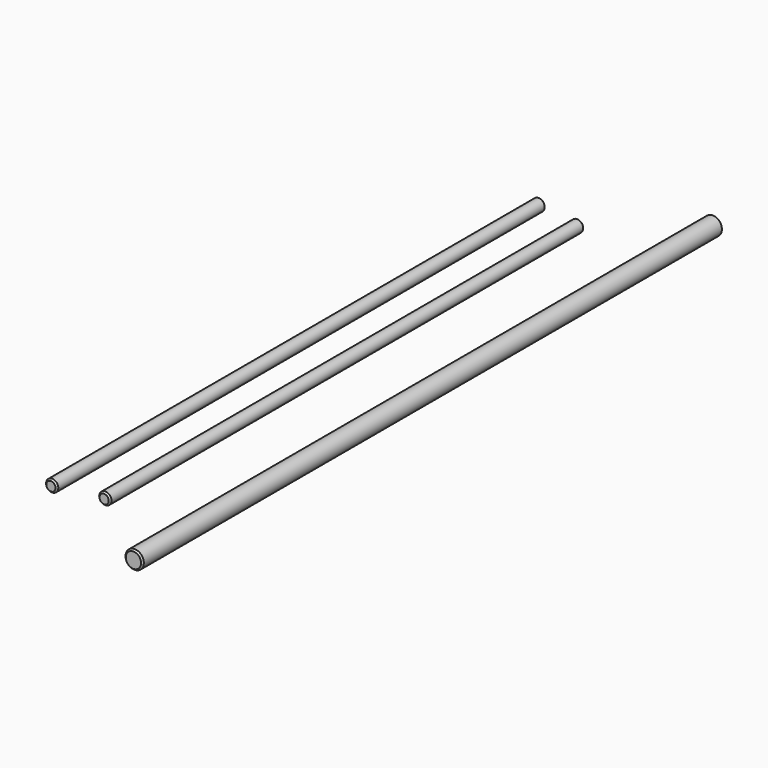
from build123d import *

# Parameters (mm, degrees)
F3_R      = 4
F4_DEPTH  = 194
F5_SIZE   = 1
F6_R      = 6
F7_DEPTH  = 237.5
F8_SIZE   = 1
F9_R      = 4
F10_DEPTH = 200
F11_SIZE  = 1


with BuildPart() as f4:
    # F3 (on Front) → F4 (new body, symmetric)
    with BuildSketch(Plane.XZ):
        with Locations((-30, 0)):
            Circle(F3_R)
    extrude(amount=F4_DEPTH, both=True)

    # F5
    f5_edges = [f4.edges().sort_by_distance(p)[0] for p in [
        (-34, -194, 0),
        (-34, 194, 0),
    ]]
    chamfer(f5_edges, length=F5_SIZE)


with BuildPart() as f7:
    # F6 (on Front) → F7 (new body, symmetric)
    with BuildSketch(Plane.XZ):
        with Locations((24, 0)):
            Circle(F6_R)
    extrude(amount=F7_DEPTH, both=True)

    # F8
    f8_edges = [f7.edges().sort_by_distance(p)[0] for p in [
        (18, -237.5, 0),
        (18, 237.5, 0),
    ]]
    chamfer(f8_edges, length=F8_SIZE)


with BuildPart() as f10:
    # F9 (on Front) → F10 (new body, symmetric)
    with BuildSketch(Plane.XZ):
        with Locations((-60, 0)):
            Circle(F9_R)
    extrude(amount=F10_DEPTH, both=True)

    # F11
    f11_edges = [f10.edges().sort_by_distance(p)[0] for p in [
        (-64, 200, 0),
        (-64, -200, 0),
    ]]
    chamfer(f11_edges, length=F11_SIZE)


solid = Compound([f4.part, f7.part, f10.part])
